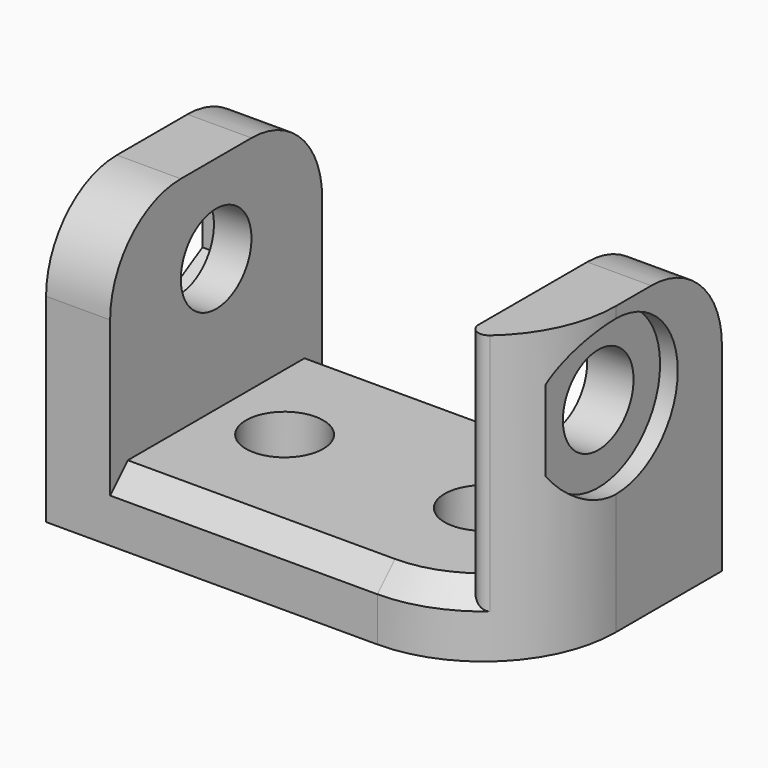
from build123d import *

# Parameters (mm, degrees)
F0_W        = 21
F0_H        = 12
F0_R        = 1.75
F1_DEPTH    = 3
F2_W        = 2.9
F2_H        = 12
F3_DEPTH    = 10
F4_R        = 2
F5_DEPTH    = 21.001
F6_T1_DEPTH = 43
F7_SIZE     = 1
F8_R        = 4
F9_R        = 0.5
F10_R       = 3.5
F11_DEPTH   = 0.8
F13_DEPTH   = 1.2


# Not quite as in the source:
# - a fillet or chamfer that OpenCascade refuses, or shapes differently, is made with other operations: its cross-section is extruded or revolved along the edge and cut away or added


with BuildPart() as f1:
    # F0 (on Top) → F1 (new body)
    with BuildSketch(Plane.XY):
        with Locations((10.5, 6)):
            Rectangle(F0_W, F0_H)
        with Locations((6, 6)):
            Circle(F0_R, mode=Mode.SUBTRACT)
        with Locations((15, 6)):
            Circle(F0_R, mode=Mode.SUBTRACT)
    extrude(amount=F1_DEPTH)

    # F2 (on face) → F3 (join)
    with BuildSketch(Plane.XY.offset(3)):
        with Locations((1.45, 6)):
            Rectangle(F2_W, F2_H)
        with Locations((19.55, 6)):
            Rectangle(F2_W, F2_H)
    extrude(amount=F3_DEPTH)

    # F4 (on face) → F5 (cut, through all)
    with BuildSketch(Plane(origin=(0, 0, 0), x_dir=(0, -1, 0), z_dir=(-1, 0, 0))):
        with Locations((-6, 9)):
            Circle(F4_R)
    extrude(amount=-F5_DEPTH, mode=Mode.SUBTRACT)

    # F6: fillet of radius 6 on 1 edges, made by hand

    # F6_s2 → F6_t1 (cut)
    with BuildSketch(Plane.XY.offset(-15)):
        with BuildLine():
            ThreePointArc((15, 0), (19.2426406871, 1.7573593129), (21, 6))
            Line((21, 6), (21, 0))
            Line((21, 0), (15, 0))
        make_face()
    extrude(amount=F6_T1_DEPTH, mode=Mode.SUBTRACT)

    # F7
    f7_edges = [f1.edges().sort_by_distance(p)[0] for p in [
        (8.95, 0, 3),
        (10.5, 12, 3),
    ]]
    chamfer(f7_edges, length=F7_SIZE)

    # F8
    f8_edges = [f1.edges().sort_by_distance(p)[0] for p in [
        (19.55, 12, 13),
        (1.45, 0, 13),
        (1.45, 12, 13),
    ]]
    fillet(f8_edges, radius=F8_R)

    # F9
    f9_edges = [f1.edges().sort_by_distance(p)[0] for p in [
        (18.1, 0.86288, 8),
    ]]
    fillet(f9_edges, radius=F9_R)

    # F10 (on face) → F11 (cut)
    with BuildSketch(Plane.YZ.offset(21)):
        with Locations((6, 9)):
            Circle(F10_R)
    extrude(amount=-F11_DEPTH, mode=Mode.SUBTRACT)

    # F12 (on face) → F13 (cut)
    with BuildSketch(Plane(origin=(0, 0, 0), x_dir=(0, -1, 0), z_dir=(-1, 0, 0))):
        Polygon((-3.15, 7.3545517328), (-3.15, 10.6454482672), (-6, 12.2908965344), (-8.85, 10.6454482672), (-8.85, 7.3545517328), (-6, 5.7091034656), align=None)
    extrude(amount=-F13_DEPTH, mode=Mode.SUBTRACT)


solid = f1.part
